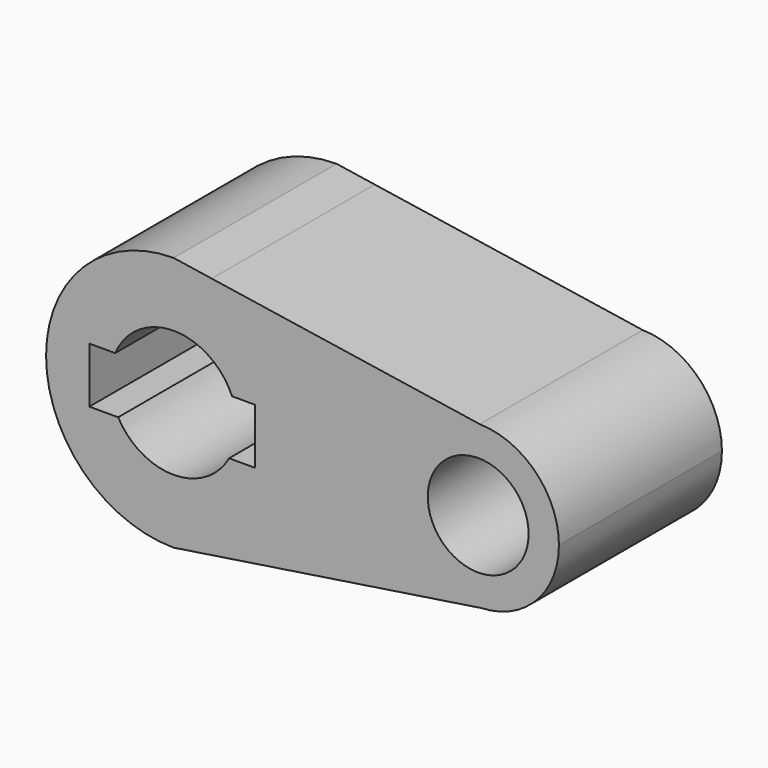
from build123d import *

# Parameters (mm, degrees)
F0_R     = 12.5710937777
F1_DEPTH = 50.8


with BuildPart() as f1:
    # F0 (on Front) → F1 (new body)
    with BuildSketch(Plane.XZ):
        with BuildLine():
            Line((9.5049608148, 30.3477681373), (0, 31.8014356752))
            ThreePointArc((0, 31.8014356752), (-31.8014356752, 0), (0, -31.8014356752))
            Line((0, -31.8014356752), (9.4712928792, -30.3582924783))
            ThreePointArc((9.4712928792, -30.3582924783), (25.6176894183, -18.8431764804), (31.8014356752, 0))
            ThreePointArc((31.8014356752, 0), (25.6281360125, 18.8289658646), (9.5049608148, 30.3477681373))
        make_face()
        with BuildLine():
            ThreePointArc((-14.5709457578, 6.1619072221), (0, 15.8202895325), (14.5709457578, 6.1619072221))
            Line((14.5709457578, 6.1619072221), (20.2656146139, 6.1619072221))
            Line((20.2656146139, 6.1619072221), (20.2656146139, -7.6786847785))
            Line((20.2656146139, -7.6786847785), (13.8318242095, -7.6786847785))
            ThreePointArc((13.8318242095, -7.6786847785), (0, -15.8202895325), (-13.8318242095, -7.6786847785))
            Line((-13.8318242095, -7.6786847785), (-21.0093853861, -7.6786847785))
            Line((-21.0093853861, -7.6786847785), (-21.0093853861, 6.1619072221))
            Line((-21.0093853861, 6.1619072221), (-14.5709457578, 6.1619072221))
        make_face(mode=Mode.SUBTRACT)
        with BuildLine():
            Line((76.3308829682, 20.1275604352), (9.5049608148, 30.3477681373))
            ThreePointArc((9.5049608148, 30.3477681373), (25.6281360125, 18.8289658646), (31.8014356752, 0))
            ThreePointArc((31.8014356752, 0), (25.6176894183, -18.8431764804), (9.4712928792, -30.3582924783))
            Line((9.4712928792, -30.3582924783), (76.6803919445, -20.1176257266))
            ThreePointArc((76.6803919445, -20.1176257266), (55.8029369519, -0.1748250718), (76.3308829682, 20.1275604352))
        make_face()
        with BuildLine():
            ThreePointArc((96.0651373404, 0), (90.3085177912, 14.0939657718), (76.3308829682, 20.1275604352))
            ThreePointArc((76.3308829682, 20.1275604352), (55.8029369519, -0.1748250718), (76.6803919445, -20.1176257266))
            ThreePointArc((76.6803919445, -20.1176257266), (90.4303700533, -13.9686006721), (96.0651373404, 0))
        make_face()
        with Locations((75.9336575866, 0)):
            Circle(F0_R, mode=Mode.SUBTRACT)
    extrude(amount=F1_DEPTH)


solid = f1.part
